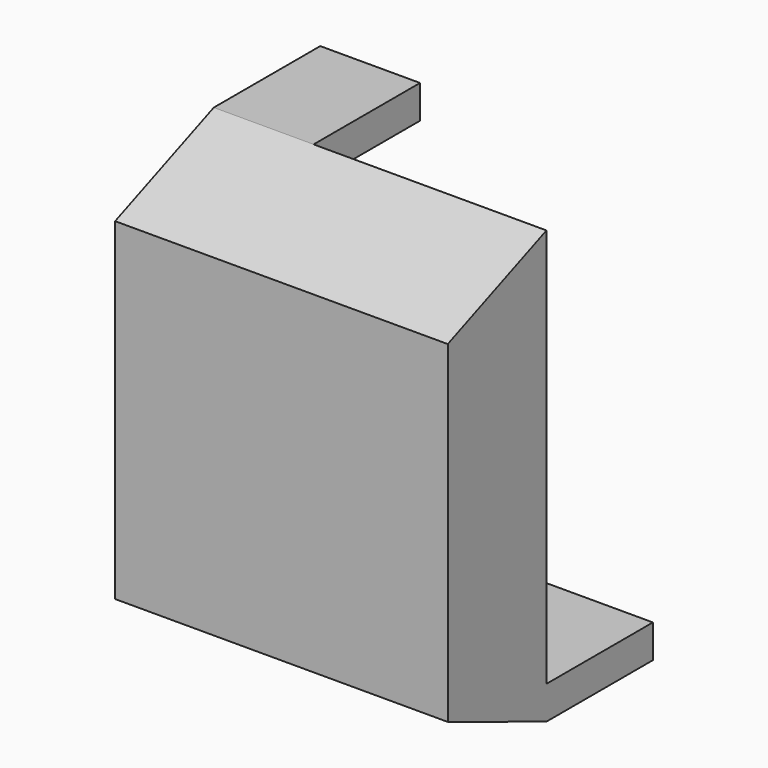
from build123d import *

# Parameters (mm, degrees)
F1_DEPTH  = 127
F0_W      = 50.8
F0_H      = 12.7
F2_DEPTH  = 38.1
F3_W      = 63.5
F3_H      = 12.7
F3_W_2    = 38.1
F4_DEPTH  = 50.8
F5_R      = 3.81
F6_DEPTH  = 50.8
F7_R      = 3.81
F8_DEPTH  = 50.8
F9_R      = 3.81
F10_DEPTH = 50.8


# Not quite as in the source:
# - a feature names something its author has since deleted; it is built from what else it names


with BuildPart() as f1:
    # F0 (on Right) → F1 (new body)
    with BuildSketch(Plane.YZ):
        Polygon((37.9020869732, -44.5222934544), (37.9020869732, 107.8777065456), (-9.1907734199, 88.8277065456), (-9.1907734199, -38.1722934544), (37.9020869732, -57.2222934544), align=None)
    extrude(amount=F1_DEPTH)

    # F0 (on Right) → F2 (join)
    with BuildSketch(Plane.YZ):
        with Locations((63.3020869732, -50.8722934544)):
            Rectangle(F0_W, F0_H)
    extrude(amount=F2_DEPTH)

    # F3 (on face) → F4 (join)
    with BuildSketch(Plane(origin=(0, 37.9020869732, 0), x_dir=(-1, 0, 0), z_dir=(0, 1, 0))):
        with Locations((-95.25, -50.8722934544)):
            Rectangle(F3_W, F3_H)
        with Locations((-19.05, 101.5277065456)):
            Rectangle(F3_W_2, F3_H)
    extrude(amount=F4_DEPTH)

    # F5 (on face) → F6 (cut)
    with BuildSketch(Plane(origin=(0, 88.7020869732, 0), x_dir=(-1, 0, 0), z_dir=(0, 1, 0))):
        with Locations((-7.62, 101.5277065456)):
            Circle(F5_R)
        with Locations((-30.48, 101.5277065456)):
            Circle(F5_R)
    extrude(amount=-F6_DEPTH, mode=Mode.SUBTRACT)

    # F7 (on face) → F8 (cut)
    with BuildSketch(Plane(origin=(0, 88.7020869732, 0), x_dir=(-1, 0, 0), z_dir=(0, 1, 0))):
        with Locations((-30.48, -50.8722934544)):
            Circle(F7_R)
        with Locations((-7.62, -50.8722934544)):
            Circle(F7_R)
    extrude(amount=-F8_DEPTH, mode=Mode.SUBTRACT)

    # F9 (on face) → F10 (cut)
    with BuildSketch(Plane(origin=(0, 88.7020869732, 0), x_dir=(-1, 0, 0), z_dir=(0, 1, 0))):
        with Locations((-71.12, -50.8722934544)):
            Circle(F9_R)
        with Locations((-119.38, -50.8722934544)):
            Circle(F9_R)
    extrude(amount=-F10_DEPTH, mode=Mode.SUBTRACT)


solid = f1.part
